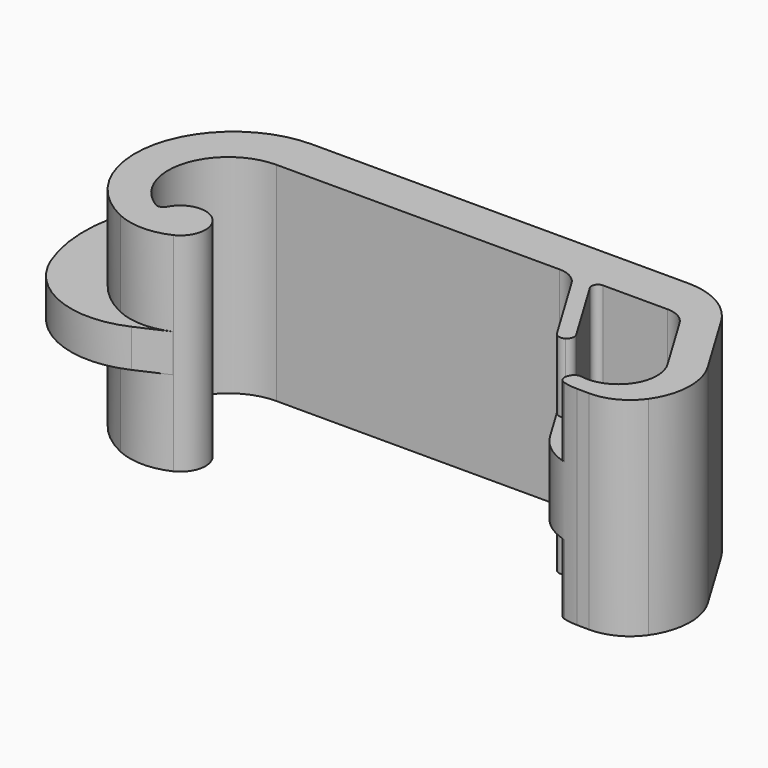
from build123d import *

# Parameters (mm, degrees)
F1_DEPTH    = 8.2
F2_DEPTH    = 1
F4_DEPTH    = 5.5
F15_DEPTH   = 5.5
F5_R        = 2
F16_R       = 0.5
F17_R       = 2
F18_R       = 5
F19_R       = 0.5
F6_R        = 0.59999
F8_DEPTH    = 8.2
F9_T1_DEPTH = 31.0823571676
F10_R       = 4
F12_DEPTH   = 1.5
F13_R       = 7


# Not quite as in the source:
# - a fillet or chamfer that OpenCascade refuses, or shapes differently, is made with other operations: its cross-section is extruded or revolved along the edge and cut away or added
# - a fillet or chamfer is up to 0.001 mm smaller than in the source, because OpenCascade refuses the exact size


with BuildPart() as f1:
    # F0 (on Top) → F1 (new body, symmetric)
    with BuildSketch(Plane.XY):
        with BuildLine():
            Line((-7.6991717756, 9.5581562555), (-40.1991717756, 9.5581562555))
            ThreePointArc((-40.1991717756, 9.5581562555), (-47.4491717756, 2.3081562555), (-40.1991717756, -4.9418437445))
            ThreePointArc((-40.1991717756, -4.9418437445), (-38.6431985652, -1.6852820196), (-42.1543481568, -2.5207911129))
            ThreePointArc((-42.1543481568, -2.5207911129), (-44.8427156809, 2.8081562555), (-40.1991717756, 6.5581562555))
            Line((-40.1991717756, 6.5581562555), (-16.7462805126, 6.5581562555))
            Line((-16.7462805126, 6.5581562555), (-11.035484998, -2.9462035475))
            ThreePointArc((-11.035484998, -2.9462035475), (-4.6547300014, -4.5371044474), (-3.0638291014, 1.8436505492))
            Line((-3.0638291014, 1.8436505492), (-7.6991717756, 9.5581562555))
        make_face()
        with BuildLine():
            Line((-15.346320436, 6.5581562555), (-8.229856713, 6.5581562555))
            Line((-8.229856713, 6.5581562555), (-4.7781637028, 0.8135743994))
            ThreePointArc((-4.7781637028, 0.8135743994), (-5.8216578415, -3.3716519963), (-10.0068842371, -2.3281578576))
            Line((-10.0068842371, -2.3281578576), (-15.346320436, 6.5581562555))
        make_face(mode=Mode.SUBTRACT)
    extrude(amount=F1_DEPTH, both=True)

    # F0 (on Top) → F2 (join, symmetric)
    with BuildSketch(Plane.XY):
        with BuildLine():
            Line((-4.7781637028, 0.8135743994), (-8.229856713, 6.5581562555))
            Line((-8.229856713, 6.5581562555), (-15.346320436, 6.5581562555))
            Line((-15.346320436, 6.5581562555), (-10.0068842371, -2.3281578576))
            ThreePointArc((-10.0068842371, -2.3281578576), (-5.8216578415, -3.3716519963), (-4.7781637028, 0.8135743994))
        make_face()
    extrude(amount=F2_DEPTH, both=True)

    # F3 (on face) → F4 (cut)
    with BuildSketch(Plane.XY.offset(8.2)):
        Polygon((-9.8084988335, -7.0643632576), (-7.0496570497, -0.5512764992), (-8.3826289276, 1.6671612479), (-13.2850058391, -1.2784839779), align=None)
    extrude(amount=-F4_DEPTH, mode=Mode.SUBTRACT)

    # F14 (on face) → F15 (cut)
    with BuildSketch(Plane(origin=(0, 0, -8.2), x_dir=(1, 0, 0), z_dir=(0, 0, -1))):
        with BuildLine():
            Line((-12.3684568759, 0.7277658005), (-11.3398561151, 0.1097201106))
            Line((-11.3398561151, 0.1097201106), (-10.0068842371, 2.3281578576))
            ThreePointArc((-10.0068842371, 2.3281578576), (-9.3022346771, 3.1354223006), (-8.3618696665, 3.649154264))
            Line((-8.3618696665, 3.649154264), (-8.8633257373, 4.8329941325))
            ThreePointArc((-8.8633257373, 4.8329941325), (-10.099006978, 4.0618270279), (-11.035484998, 2.9462035475))
            Line((-11.035484998, 2.9462035475), (-12.3684568759, 0.7277658005))
        make_face()
    extrude(amount=-F15_DEPTH, mode=Mode.SUBTRACT)

    # F5
    f5_edges = [f1.edges().sort_by_distance(p)[0] for p in [
        (-16.746281, 6.558156, 0),
    ]]
    fillet(f5_edges, radius=F5_R)

    # F16
    f16_edges = [f1.edges().sort_by_distance(p)[0] for p in [
        (-15.34632, 6.558156, -4.6),
        (-15.34632, 6.558156, 4.6),
    ]]
    fillet(f16_edges, radius=F16_R)

    # F17
    f17_edges = [f1.edges().sort_by_distance(p)[0] for p in [
        (-8.229857, 6.558156, -4.6),
        (-8.229857, 6.558156, 4.6),
    ]]
    fillet(f17_edges, radius=F17_R)

    # F18
    f18_edges = [f1.edges().sort_by_distance(p)[0] for p in [
        (-7.699172, 9.558156, 0),
    ]]
    fillet(f18_edges, radius=F18_R)

    # F19
    f19_edges = [f1.edges().sort_by_distance(p)[0] for p in [
        (-42.154348, -2.520791, 0),
    ]]
    fillet(f19_edges, radius=F19_R)

    # F6 (radius 0.6 in the source; OpenCascade refuses exactly that, so slightly less here)
    f6_edges = [f1.edges().sort_by_distance(p)[0] for p in [
        (-12.368457, -0.727766, 5.45),
        (-11.339856, -0.10972, 5.45),
        (-8.36187, -3.649154, 5.45),
        (-8.863326, -4.832994, 5.45),
        (-8.863326, -4.832994, -5.45),
        (-8.36187, -3.649154, -5.45),
        (-12.368457, -0.727766, -5.45),
        (-11.339856, -0.10972, -5.45),
    ]]
    fillet(f6_edges, radius=F6_R)

    # F7 (on Top) → F8 (join, symmetric)
    with BuildSketch(Plane.XY):
        with BuildLine():
            ThreePointArc((-40.1991717756, -4.9418437445), (-47.4491717756, 2.3081562555), (-40.1991717756, 9.5581562555))
            Line((-40.1991717756, 9.5581562555), (-10.5280356666, 9.5581562555))
            ThreePointArc((-10.5280356666, 9.5581562555), (-8.065917866, 8.9099347352), (-6.242199163, 7.13334663))
            Line((-6.242199163, 7.13334663), (-3.0638291014, 1.8436505492))
            ThreePointArc((-3.0638291014, 1.8436505492), (-3.0131583432, -2.8597777863), (-7.0927569488, -5.2010767528))
            Line((-7.0927569488, -5.2010767528), (-4.8792576743, -5.2215941063))
            ThreePointArc((-4.8792576743, -5.2215941063), (-2.1256697511, -2.0601996528), (-2.6352454511, 2.1011695866))
            Line((-2.6352454511, 2.1011695866), (-5.8136155127, 7.3908656675))
            ThreePointArc((-5.8136155127, 7.3908656675), (-7.819706086, 9.3451125832), (-10.5280356666, 10.0581562555))
            Line((-10.5280356666, 10.0581562555), (-40.1991717756, 10.0581562555))
            ThreePointArc((-40.1991717756, 10.0581562555), (-47.9456545804, 2.5416175049), (-40.6658823702, -5.4277781561))
            Line((-40.6658823702, -5.4277781561), (-39.2876185276, -4.7220321267))
            ThreePointArc((-39.2876185276, -4.7220321267), (-39.7303310587, -4.8861144001), (-40.1991717756, -4.9418437445))
        make_face()
    extrude(amount=F8_DEPTH, both=True)

    # F9: fillet of radius 5 on 1 edges, made by hand

    # F9_s2 → F9_t1 (cut)
    with BuildSketch(Plane.XY.offset(-15.5411785838)):
        with BuildLine():
            ThreePointArc((-39.2876185276, -4.7220321267), (-41.4015983231, -5.1781218435), (-43.5104409693, -4.6988399859))
            Line((-43.5104409693, -4.6988399859), (-43.5531670234, -4.7892528406))
            ThreePointArc((-43.5531670234, -4.7892528406), (-42.1478250371, -5.2961353267), (-40.6719044424, -5.5275966647))
            Line((-40.6719044424, -5.5275966647), (-40.6203047078, -5.5167875752))
            ThreePointArc((-40.6203047078, -5.5167875752), (-39.9311727865, -5.1639145605), (-39.2458881329, -4.8129088242))
            Line((-39.2458881329, -4.8129088242), (-39.2876185276, -4.7220321267))
        make_face()
    extrude(amount=F9_T1_DEPTH, mode=Mode.SUBTRACT)

    # F10
    f10_edges = [f1.edges().sort_by_distance(p)[0] for p in [
        (-4.879258, -5.221594, 0),
    ]]
    fillet(f10_edges, radius=F10_R)

    # F11 (on Top) → F12 (join, symmetric)
    with BuildSketch(Plane.XY):
        with BuildLine():
            Line((-9.8019854711, 10.0100230104), (-40.1991717756, 14.0581562555))
            ThreePointArc((-40.1991717756, 14.0581562555), (-51.5354352526, 5.3987274618), (-46.1626661567, -7.8160343179))
            Line((-46.1626661567, -7.8160343179), (-39.3222752617, -4.7377869483))
            ThreePointArc((-39.3222752617, -4.7377869483), (-41.4206326973, -5.1779810716), (-43.5104409693, -4.6988399859))
            ThreePointArc((-43.5104409693, -4.6988399859), (-47.7611398022, 4.0049590032), (-40.1991717756, 10.0581562555))
            Line((-40.1991717756, 10.0581562555), (-10.5280356666, 10.0581562555))
            ThreePointArc((-10.5280356666, 10.0581562555), (-10.1642136992, 10.0461097517), (-9.8019854711, 10.0100230104))
        make_face()
    extrude(amount=F12_DEPTH, both=True)

    # F13
    f13_edges = [f1.edges().sort_by_distance(p)[0] for p in [
        (-46.162666, -7.816034, 0),
    ]]
    fillet(f13_edges, radius=F13_R)


solid = f1.part
